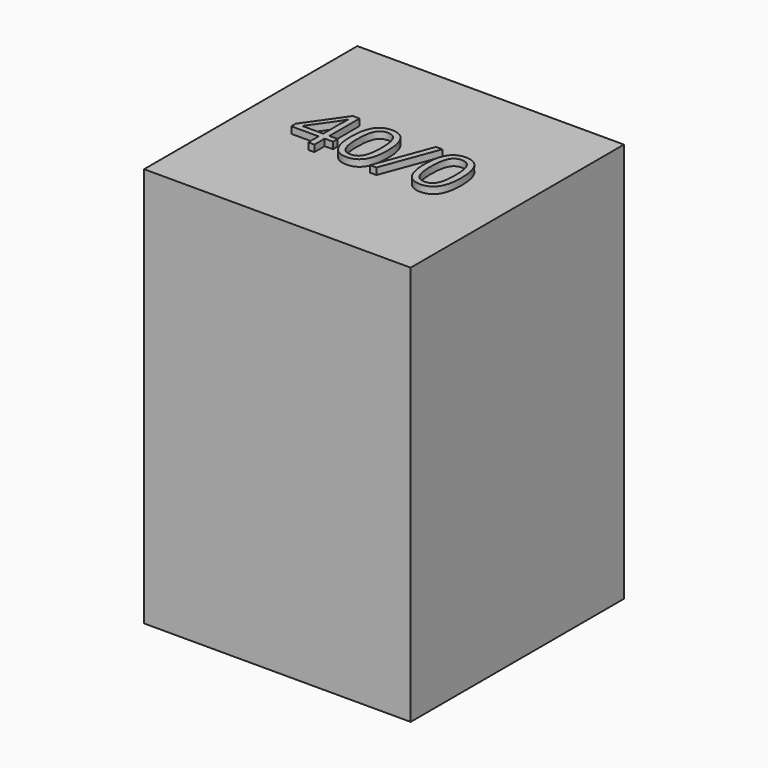
from build123d import *

# Parameters (mm, degrees)
F0_W         = 40
F0_H         = 40
F1_DEPTH     = 60
F2_TEXT_SIZE = 11.8055555556
F3_DEPTH     = 1


# Not quite as in the source:
# - Text() gives the source's letters only with a copy of the font that has no kerning and outlines rounded to 1/6400 em; it was checked with that copy


with BuildPart() as f1:
    # F0 (on Top) → F1 (new body)
    with BuildSketch(Plane.XY):
        Rectangle(F0_W, F0_H)
    extrude(amount=F1_DEPTH)

    # F2 (on face) → F3 (join)
    with BuildSketch(Plane.XY.offset(60)):
        with Locations((-12.3810763889, -4.1591675137)):
            Text('40/0', F2_TEXT_SIZE, font='Open Sans', text_align=(TextAlign.LEFT, TextAlign.BOTTOM))
    extrude(amount=F3_DEPTH)


solid = f1.part
